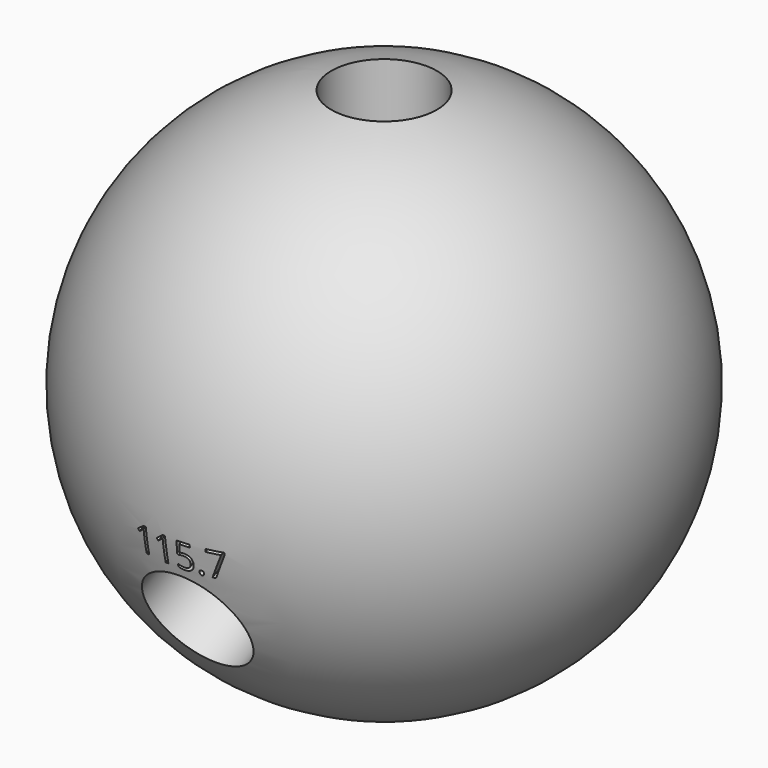
from build123d import *

# Parameters (mm, degrees)
F4_R          = 3.175
F5_DEPTH      = 50.8
F7_ANGLE      = 115.7
F8_ANGLE      = -133.8
F10_TEXT_SIZE = 2.141132912
F11_DEPTH     = 6.35
F13_TEXT_SIZE = 2.7430867906
F14_DEPTH     = 6.35


# Not quite as in the source:
# - Text() gives the source's letters only with a copy of the font that has no kerning and outlines rounded to 1/6400 em; it was checked with that copy


with BuildPart() as f2:
    # F0 (on Front) → F2 (revolve)
    with BuildSketch(Plane.XZ):
        with BuildLine():
            Line((0, -15.875), (0, 15.875))
            ThreePointArc((0, 15.875), (-15.875, 0), (0, -15.875))
        make_face()
    revolve(axis=Axis((0, 0, 0), (0, 0, 1)))

    # F10 (on offset) → F11 (cut)
    with BuildSketch(Plane(origin=(0, -17.1655172562, -8.2612055614), x_dir=(1, 0, 0), z_dir=(0, -0.9010770213, -0.4336590846))):
        with Locations((-2.5474213762, 3.6634134594)):
            Text('115.7', F10_TEXT_SIZE, font='Open Sans', text_align=(TextAlign.LEFT, TextAlign.BOTTOM))
    extrude(amount=-F11_DEPTH, mode=Mode.SUBTRACT)

    # F13 (on offset) → F14 (cut)
    with BuildSketch(Plane(origin=(0, 13.7495323453, -13.1853274622), x_dir=(-1, 0, 0), z_dir=(0, 0.7217602281, -0.6921431739))):
        with Locations((-3.3499536803, 3.8738998119)):
            Text('133.8', F13_TEXT_SIZE, font='Open Sans', text_align=(TextAlign.LEFT, TextAlign.BOTTOM))
    extrude(amount=-F14_DEPTH, mode=Mode.SUBTRACT)


with BuildPart() as f5:
    # F4 (on offset) → F5 (new body)
    with BuildSketch(Plane.XY.offset(6.35)):
        Circle(F4_R)
    extrude(amount=F5_DEPTH)


with BuildPart() as f7_1:
    # F7: copy of F5
    add(f5.part.rotate(Axis((29.5889526606, 0, 0), (1, 0, 0)), F7_ANGLE))


with BuildPart() as f8_1:
    # F8: copy of F5
    add(f5.part.rotate(Axis((29.5889526606, 0, 0), (1, 0, 0)), F8_ANGLE))


with BuildPart() as f2_1:
    add(f2.part)

    # F15: cut F5, F7_1, F8_1
    add(f5.part, mode=Mode.SUBTRACT)
    add(f7_1.part, mode=Mode.SUBTRACT)
    add(f8_1.part, mode=Mode.SUBTRACT)


solid = f2_1.part
